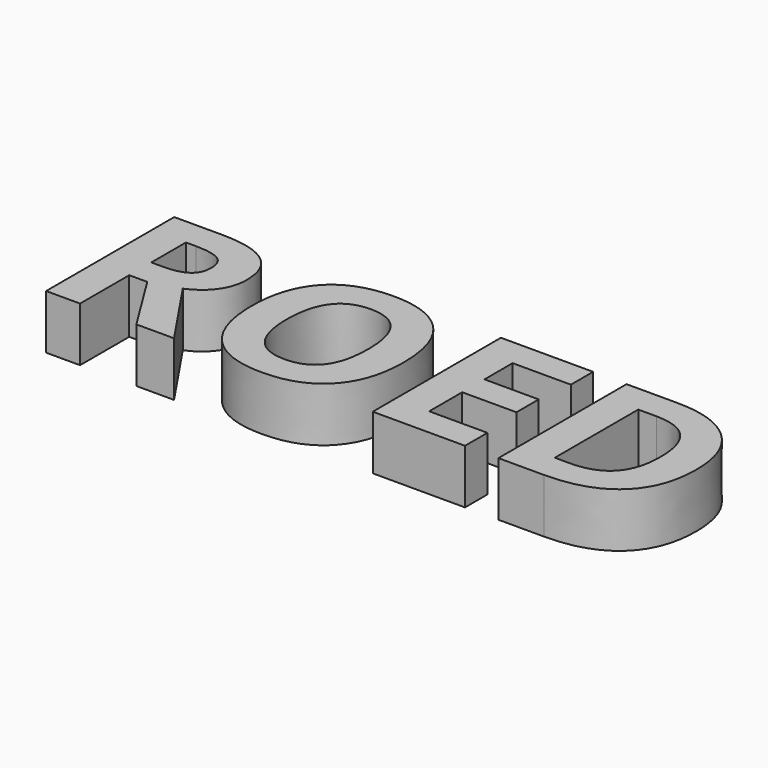
from build123d import *

# Parameters (mm, degrees)
F0_TEXT_SIZE = 52.4976316632
F1_DEPTH     = 12.7


# Not quite as in the source:
# - Text() gives the source's letters only with a copy of the font that has no kerning and outlines rounded to 1/6400 em; it was checked with that copy


with BuildPart() as f1:
    # F0 (on Top) → F1 (new body)
    with BuildSketch(Plane.XY):
        with Locations((-53.9873950183, -45.9072478116)):
            Text('ROED', F0_TEXT_SIZE, font='Open Sans', font_style=FontStyle.BOLD, text_align=(TextAlign.LEFT, TextAlign.BOTTOM))
    extrude(amount=F1_DEPTH)


solid = f1.part
